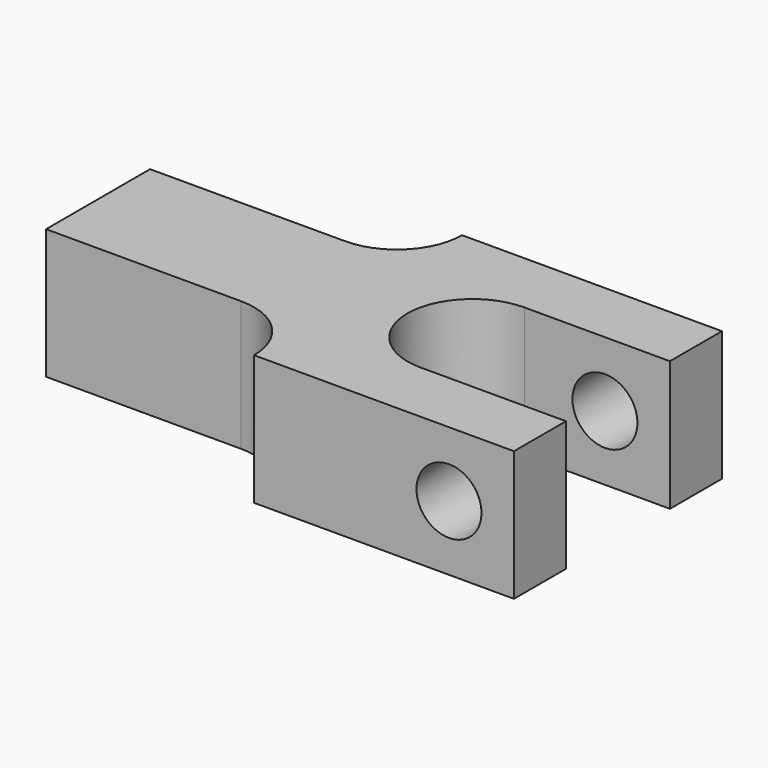
from build123d import *

# Parameters (mm, degrees)
F1_DEPTH = 3.175
F2_R     = 3.17499
F4_D     = 3.175
F6_D     = 4.0386
F6_DEPTH = 13.462
F6_TIP   = 1.213317848


# Not quite as in the source:
# - a fillet or chamfer is up to 0.001 mm smaller than in the source, because OpenCascade refuses the exact size


with BuildPart() as f1:
    # F0 (on Top) → F1 (new body, symmetric)
    with BuildSketch(Plane.XY):
        with BuildLine():
            Line((-5.588, -3.175), (-5.588, -6.35))
            Line((-5.588, -6.35), (7.112, -6.35))
            Line((7.112, -6.35), (7.112, -3.175))
            Line((7.112, -3.175), (0, -3.175))
            ThreePointArc((0, -3.175), (-3.175, 0), (0, 3.175))
            Line((0, 3.175), (7.112, 3.175))
            Line((7.112, 3.175), (7.112, 6.35))
            Line((7.112, 6.35), (-5.588, 6.35))
            Line((-5.588, 6.35), (-5.588, 3.175))
            Line((-5.588, 3.175), (-18.288, 3.175))
            Line((-18.288, 3.175), (-18.288, -3.175))
            Line((-18.288, -3.175), (-5.588, -3.175))
        make_face()
    extrude(amount=F1_DEPTH, both=True)

    # F2 (radius 3.175 in the source; OpenCascade refuses exactly that, so slightly less here)
    f2_edges = [f1.edges().sort_by_distance(p)[0] for p in [
        (-5.588, -3.175, 0),
        (-5.588, 3.175, 0),
    ]]
    fillet(f2_edges, radius=F2_R)

    # F4 (through all)
    with Locations(Plane.XZ.offset(6.35)):
        with Locations((3.937, 0)):
            Hole(F4_D / 2)

    # F6
    with Locations(Plane(origin=(-18.288, 0, 0), x_dir=(0, -1, 0), z_dir=(-1, 0, 0))):
        with Locations((0, 0)):
            Hole(F6_D / 2, depth=F6_DEPTH)
            with Locations((0, 0, -(F6_DEPTH + F6_TIP / 2))):  # 118° drill point
                Cone(0, F6_D / 2, F6_TIP, mode=Mode.SUBTRACT)


solid = f1.part
